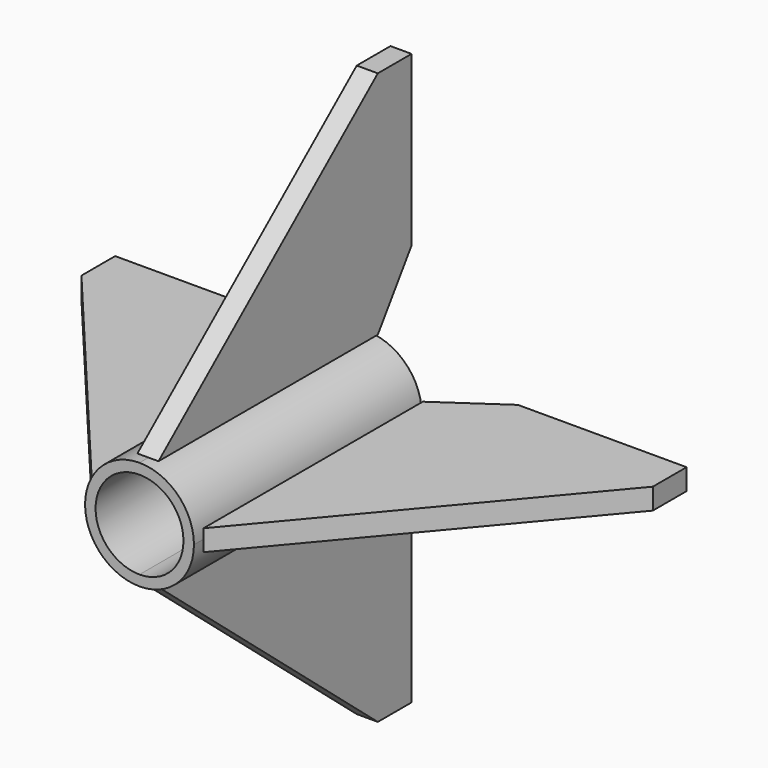
from build123d import *

# Parameters (mm, degrees)
F1_DEPTH = 171.45
F3_DEPTH = 6.35
F5_DEPTH = 6.35
F7_DEPTH = 38.1


# Not quite as in the source:
# - a feature names something its author has since deleted; it is built from what else it names


with BuildPart() as f1:
    # F0 (on Front) → F1 (new body)
    with BuildSketch(Plane.XZ):
        with BuildLine():
            ThreePointArc((0, -32.7790447839), (23.1782848475, -23.1782848475), (32.7790447839, 0))
            ThreePointArc((32.7790447839, 0), (23.1782848475, 23.1782848475), (0, 32.7790447839))
            Line((0, 32.7790447839), (0, 26.4696761765))
            ThreePointArc((0, 26.4696761765), (18.7168875202, 18.7168875202), (26.4696761765, 0))
            ThreePointArc((26.4696761765, 0), (18.7168875202, -18.7168875202), (0, -26.4696761765))
            Line((0, -26.4696761765), (0, -32.7790447839))
        make_face()
        with BuildLine():
            Line((0, 26.4696761765), (0, 32.7790447839))
            ThreePointArc((0, 32.7790447839), (-32.7790447839, 0), (0, -32.7790447839))
            Line((0, -32.7790447839), (0, -26.4696761765))
            ThreePointArc((0, -26.4696761765), (-26.4696761765, 0), (0, 26.4696761765))
        make_face()
    extrude(amount=F1_DEPTH)


with BuildPart() as f3:
    # F2 (on Right) → F3 (new body, symmetric)
    with BuildSketch(Plane.YZ):
        Polygon((0, -33.7008051574), (-165.1, -33.7008051574), (0, -172.2361542648), (25.4, -172.2361542648), (25.4, -70.6361542648), align=None)
    extrude(amount=F3_DEPTH, both=True)


with BuildPart() as f3b:
    # F2 (on Right) → F3, piece 2 (new body, symmetric)
    with BuildSketch(Plane.YZ):
        Polygon((0, 171.6016080213), (-165.1, 33.0662589139), (0, 33.0662589139), align=None)
        Polygon((25.4, 171.6016080213), (0, 171.6016080213), (0, 33.0662589139), (25.4, 70.0016080213), align=None)
    extrude(amount=F3_DEPTH, both=True)


with BuildPart() as f5:
    # F4 (on Top) → F5 (new body, symmetric)
    with BuildSketch(Plane.XY):
        Polygon((70.3748299711, 25.4), (33.4335446524, 0), (171.9748299711, 0), (171.9748299711, 25.4), align=None)
        Polygon((33.4335446524, 0), (33.4251142079, -165.0999997848), (171.9748299711, 0), align=None)
    extrude(amount=F5_DEPTH, both=True)


with BuildPart() as f5b:
    # F4 (on Top) → F5, piece 2 (new body, symmetric)
    with BuildSketch(Plane.XY):
        Polygon((-172.14276502, 25.4), (-172.14276502, 0), (-33.6014797013, 0), (-70.54276502, 25.4), align=None)
        Polygon((-172.14276502, 0), (-33.5930492568, -165.0999997848), (-33.6014797013, 0), align=None)
    extrude(amount=F5_DEPTH, both=True)


with BuildPart() as f7:
    # F0 (on Front) → F7 (new body)
    with BuildSketch(Plane.XZ):
        with BuildLine():
            ThreePointArc((26.4696761765, 0), (18.7168875202, 18.7168875202), (0, 26.4696761765))
            Line((0, 26.4696761765), (0, 13.8590905917))
            ThreePointArc((0, 13.8590905917), (9.7998569385, 9.7998569385), (13.8590905917, 0))
            ThreePointArc((13.8590905917, 0), (9.7998569385, -9.7998569385), (0, -13.8590905917))
            Line((0, -13.8590905917), (0, -26.4696761765))
            ThreePointArc((0, -26.4696761765), (18.7168875202, -18.7168875202), (26.4696761765, 0))
        make_face()
        with BuildLine():
            Line((0, 13.8590905917), (0, 26.4696761765))
            ThreePointArc((0, 26.4696761765), (-26.4696761765, 0), (0, -26.4696761765))
            Line((0, -26.4696761765), (0, -13.8590905917))
            ThreePointArc((0, -13.8590905917), (-13.8590905917, 0), (0, 13.8590905917))
        make_face()
    extrude(amount=F7_DEPTH)


solid = Compound([f1.part, f3.part, f3b.part, f5.part, f5b.part, f7.part])
